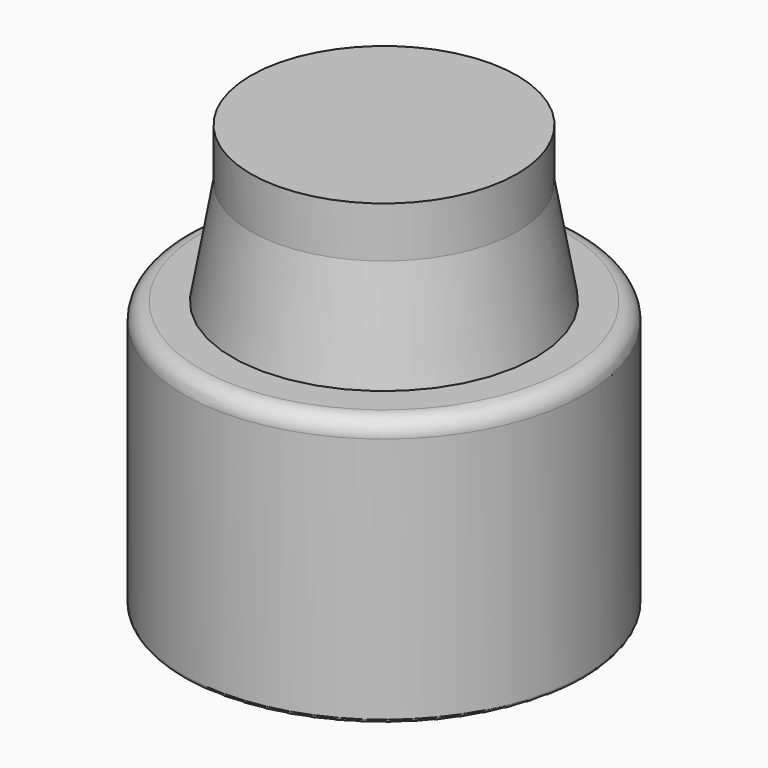
from build123d import *

# Parameters (mm, degrees)
F2_R     = 10.845
F3_DEPTH = 15.8
F4_R     = 8.15
F5_DEPTH = 1
F5_TAPER = 80


# Not quite as in the source:
# - an extrude ends at something that could not be found from the text; its depth is read off the source's solid


with BuildPart() as f1:
    # F0 (on Front) → F1 (revolve)
    with BuildSketch(Plane.XZ):
        with BuildLine():
            Line((10.845, 15.8), (8.15, 15.8))
            Line((8.15, 15.8), (8.15, 7.4))
            Line((8.15, 7.4), (1.5, 3.5606207099))
            Line((1.5, 3.5606207099), (0, 3.5606207099))
            Line((0, 3.5606207099), (0, 0))
            Line((0, 0), (11.65, 0))
            ThreePointArc((11.65, 0), (11.7878858223, 0.0571141777), (11.845, 0.195))
            Line((11.845, 0.195), (11.845, 14.8))
            ThreePointArc((11.845, 14.8), (11.5521067812, 15.5071067812), (10.845, 15.8))
        make_face()
    revolve(axis=Axis((0, 0, 1.7803103549), (0, 0, -1)))

    # F2 (on face) → F3 (join, through all)
    with BuildSketch(Plane.XY.offset(15.8)):
        Circle(F2_R)
        Polygon((-8.2041473252, 0), (-4.1020736626, 7.105), (4.1020736626, 7.105), (8.2041473252, 0), (4.1020736626, -7.105), (-4.1020736626, -7.105), align=None, mode=Mode.SUBTRACT)
    extrude(amount=-F3_DEPTH)

    # F4 (on face) → F5 (cut)
    with BuildSketch(Plane.XY.offset(15.8)):
        Circle(F4_R)
    extrude(amount=-F5_DEPTH, taper=F5_TAPER, mode=Mode.SUBTRACT)


with BuildPart() as f7:
    # F6 (on Front) → F7 (revolve)
    with BuildSketch(Plane.XZ):
        with BuildLine():
            Line((7.875, 25), (0, 25))
            Line((0, 25), (0, 0))
            Line((0, 0), (7.865, 0))
            Line((7.865, 0), (9.3503139047, 8.4236337441))
            ThreePointArc((9.3503139047, 8.4236337441), (9.5781976095, 11.0283564091), (9.3503139047, 13.6330790741))
            Line((9.3503139047, 13.6330790741), (7.875, 22))
            Line((7.875, 22), (7.875, 25))
        make_face()
    revolve(axis=Axis((0, 0, 12.5), (0, 0, -1)))


with BuildPart() as f9:
    # F8 (on Front) → F9 (revolve)
    with BuildSketch(Plane.XZ):
        with BuildLine():
            Line((0, 7.0269373127), (0, 0))
            Line((0, 0), (5.3425146232, 0))
            ThreePointArc((5.3425146232, 0), (5.679504679, 0.1306252549), (5.840417087, 0.4542491907))
            Line((5.840417087, 0.4542491907), (6.2935137888, 5.3852650008))
            ThreePointArc((6.2935137888, 5.3852650008), (6.3100029903, 6.2569191501), (6.2, 7.1217614432))
            ThreePointArc((6.2, 7.1217614432), (6.0365510119, 7.4013445877), (5.7360583301, 7.522118983))
            Line((5.7360583301, 7.522118983), (4.25, 7.6))
            Line((4.25, 7.6), (1, 7.0269373127))
            Line((1, 7.0269373127), (0, 7.0269373127))
        make_face()
    revolve(axis=Axis((0, 0, 3.5134686563), (0, 0, 1)))


solid = Compound([f1.part, f7.part, f9.part])
